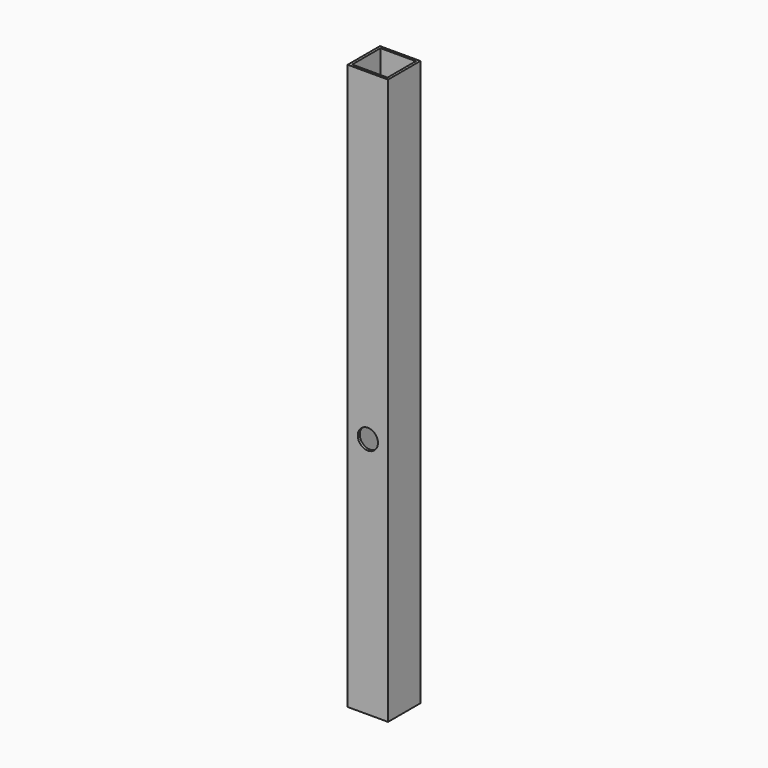
from build123d import *

# Parameters (mm, degrees)
F1_W     = 25.4
F1_H     = 25.4
F2_DEPTH = 355.6
F3_T     = -1.5875
F4_DEPTH = 1.5885
F5_R     = 6.35
F6_DEPTH = 25.401


# Not quite as in the source:
# - a variable given as a bare number and used for a length is read in inches; the dataset says mm whatever the document's units were


with BuildPart() as f2:
    # F1 (on Top) → F2 (new body)
    with BuildSketch(Plane.XY):
        Rectangle(F1_W, F1_H)
    extrude(amount=F2_DEPTH)

    # F3
    f3_openings = [f2.faces().sort_by_distance(p)[0] for p in [
        (0, 0, 355.6),
    ]]
    offset(amount=F3_T, openings=f3_openings)

    # F4 (cut, through all): a face of the model
    f4_faces = [f2.faces().sort_by_distance(p)[0] for p in [
        (0, 0, 1.5875),
    ]]
    extrude(f4_faces, amount=-F4_DEPTH, mode=Mode.SUBTRACT)

    # F5 (on face) → F6 (cut, through all)
    with BuildSketch(Plane.XZ.offset(12.7)):
        with Locations((0, 152.4)):
            Circle(F5_R)
    extrude(amount=-F6_DEPTH, mode=Mode.SUBTRACT)


solid = f2.part
